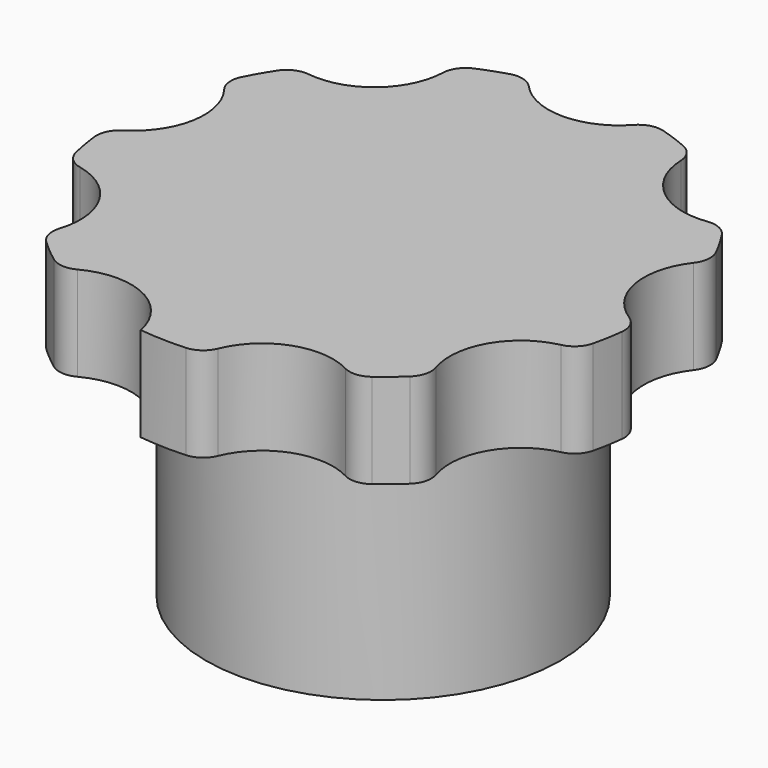
from build123d import *

# Parameters (mm, degrees)
F0_R     = 15
F0_R_2   = 11
F1_DEPTH = 20
F2_R     = 22.5
F3_DEPTH = 8
F4_R     = 6
F5_DEPTH = 25
F6_R     = 2


with BuildPart() as f1:
    # F0 (on Top) → F1 (new body)
    with BuildSketch(Plane.XY):
        Circle(F0_R)
        Circle(F0_R_2, mode=Mode.SUBTRACT)
    extrude(amount=F1_DEPTH)

    # F2 (on face) → F3 (join)
    with BuildSketch(Plane.XY.offset(20)):
        Circle(F2_R)
    extrude(amount=F3_DEPTH)

    # F4 (on face) → F5 (cut)
    with BuildSketch(Plane.XY.offset(28)):
        with Locations((0, 25)):
            Circle(F4_R)
        with Locations((-16.0696902422, 19.151111078)):
            Circle(F4_R)
        with Locations((-24.6201938253, 4.3412044417)):
            Circle(F4_R)
        with Locations((-21.6506350946, -12.5)):
            Circle(F4_R)
        with Locations((-8.5505035831, -23.4923155196)):
            Circle(F4_R)
        with Locations((8.5505035831, -23.4923155196)):
            Circle(F4_R)
        with Locations((21.6506350946, -12.5)):
            Circle(F4_R)
        with Locations((24.6201938253, 4.3412044417)):
            Circle(F4_R)
        with Locations((16.0696902422, 19.151111078)):
            Circle(F4_R)
    extrude(amount=-F5_DEPTH, mode=Mode.SUBTRACT)

    # F6
    f6_edges = [f1.edges().sort_by_distance(p)[0] for p in [
        (-16.40022, -15.403986, 24),
        (-21.540353, -6.501014, 24),
        (-22.464789, -1.25828, 24),
        (-20.679639, 8.865807, 24),
        (-18.017833, 13.476189, 24),
        (-10.142692, 20.084218, 24),
        (-5.140134, 21.905, 24),
        (5.140134, 21.905, 24),
        (18.017833, 13.476189, 24),
        (10.142692, 20.084218, 24),
        (20.679639, 8.865807, 24),
        (22.464789, -1.25828, 24),
        (21.540353, -6.501014, 24),
        (16.40022, -15.403986, 24),
        (12.322097, -18.825938, 24),
        (2.661805, -22.341996, 24),
        (-12.322097, -18.825938, 24),
    ]]
    fillet(f6_edges, radius=F6_R)


solid = f1.part
